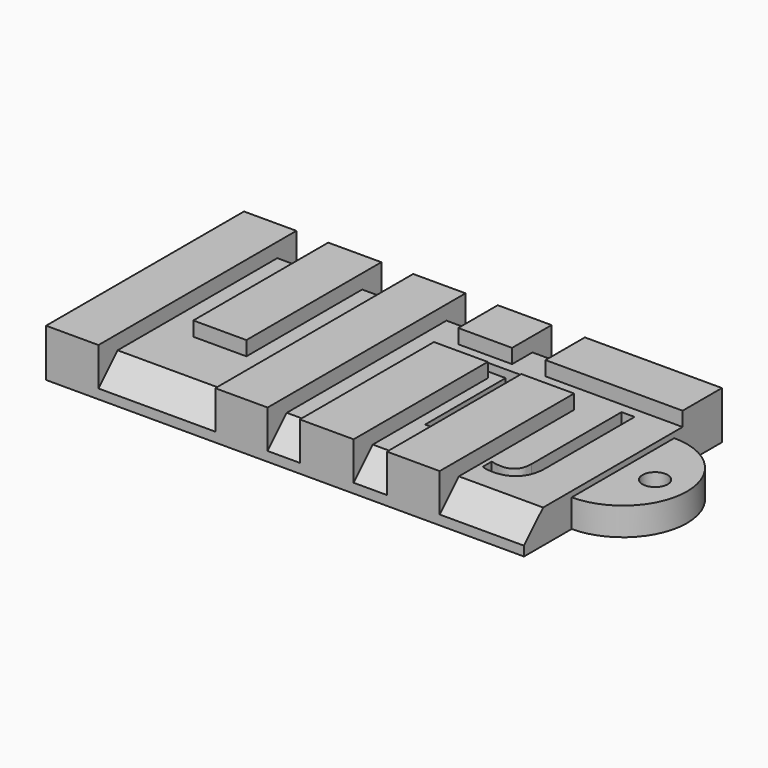
from build123d import *

# Parameters (mm, degrees)
F1_DEPTH     = 4.2
F0_W         = 6.5777550638
F0_H         = 31.0568130806
F0_W_2       = 6.6643171012
F0_H_2       = 21.1724707555
F0_W_3       = 6.5723955631
F0_W_4       = 6.7562386394
F0_H_3       = 6.1960610162
F0_H_4       = 21.0460054386
F0_W_5       = 6.6203959286
F0_H_5       = 21.0919662077
F0_W_6       = 17.2071668506
F0_H_6       = 6.1697455656
F2_DEPTH     = 6
F0_R         = 1.5875
F3_DEPTH     = 3.5
F4_TEXT_SIZE = 19.7454847188
F5_DEPTH     = 25
F6_SIZE      = 3


# Not quite as in the source:
# - Text() gives the source's letters only with a copy of the font that has no kerning and outlines rounded to 1/6400 em; it was checked with that copy


with BuildPart() as f1:
    # F0 (on Top) → F1 (new body)
    with BuildSketch(Plane.XY):
        Polygon((-63.7559369206, -7.0417550277), (-67.7545294166, -7.0417550277), (-67.7545294166, -38.0985681083), (-53.0930310488, -38.0985681083), (-53.0930310488, -7.0417550277), (-57.0916198194, -7.0417550277), (-57.0916198194, -28.2142257832), (-63.7559369206, -28.2142257832), align=None)
    extrude(amount=F1_DEPTH)



with BuildPart() as f1b:
    # F0 (on Top) → F1, piece 2 (new body)
    with BuildSketch(Plane.XY):
        Polygon((-46.5206354856, -7.0417550277), (-46.5206354856, -38.0985681083), (-42.4760840833, -38.0985681083), (-42.4760840833, -17.0525626697), (-35.719845444, -17.0525626697), (-35.719845444, -38.0985681083), (-31.5394513309, -38.0985681083), (-31.5394513309, -17.0066019006), (-24.9190554023, -17.0066019006), (-24.9190554023, -38.0985681083), (-14.3322844803, -38.0985681083), (-14.3322844803, -30.6171796859), (-14.3322844803, -14.5231434501), (-14.3322844803, -13.2115005933), (-31.5394513309, -13.2115005933), (-31.5394513309, -7.0417550277), (-35.719845444, -7.0417550277), (-35.719845444, -13.2378160439), (-42.4760840833, -13.2378160439), (-42.4760840833, -7.0417550277), align=None)
    extrude(amount=F1_DEPTH)


with BuildPart() as f1_1:
    add(f1.part)

    add(f1b.part)  # F2 merges F1b
    # F0 (on Top) → F2 (join)
    with BuildSketch(Plane.XY):
        with Locations((-71.0434069484, -22.570161568)):
            Rectangle(F0_W, F0_H)
        with Locations((-60.42377837, -17.6279904054)):
            Rectangle(F0_W_2, F0_H_2)
        with Locations((-49.8068332672, -22.570161568)):
            Rectangle(F0_W_3, F0_H)
        with Locations((-39.0979647636, -10.1397855358)):
            Rectangle(F0_W_4, F0_H_3)
        with Locations((-39.0979647636, -27.575565389)):
            Rectangle(F0_W_4, F0_H_4)
        with Locations((-28.2292533666, -27.5525850045)):
            Rectangle(F0_W_5, F0_H_5)
        with Locations((-22.9358679056, -10.1266278105)):
            Rectangle(F0_W_6, F0_H_6)
    extrude(amount=F2_DEPTH)

    # F0 (on Top) → F3 (join)
    with BuildSketch(Plane.XY):
        with BuildLine():
            Line((-14.3322844803, -14.5231434501), (-14.3322844803, -30.6171796859))
            ThreePointArc((-14.3322844803, -30.6171796859), (-6.2852663624, -22.570161568), (-14.3322844803, -14.5231434501))
        make_face()
        with Locations((-10.300190188, -22.570161568)):
            Circle(F0_R, mode=Mode.SUBTRACT)
    extrude(amount=F3_DEPTH)

    # F4 (on face) → F5 (cut)
    with BuildSketch(Plane.XY.offset(4.2)):
        with Locations((-39.0060693026, -28.5764010325)):
            Text('T', F4_TEXT_SIZE, font='Open Sans', text_align=(TextAlign.LEFT, TextAlign.BOTTOM))
        with Locations((-22.8147171438, -28.5764010325)):
            Text('J', F4_TEXT_SIZE, font='Open Sans', text_align=(TextAlign.LEFT, TextAlign.BOTTOM))
    extrude(amount=-F5_DEPTH, mode=Mode.SUBTRACT)

    # F6
    f6_edges = [f1_1.edges().sort_by_distance(p)[0] for p in [
        (-65.755233, -7.041755, 4.2),
        (-55.092325, -7.041755, 4.2),
        (-44.49836, -7.041755, 4.2),
        (-33.629648, -7.041755, 4.2),
        (-60.42378, -38.098568, 4.2),
        (-44.49836, -38.098568, 4.2),
        (-33.629648, -38.098568, 4.2),
        (-19.62567, -38.098568, 4.2),
    ]]
    chamfer(f6_edges, length=F6_SIZE)


with BuildPart() as f1_2:
    # F8: moved
    add(f1_1.part.moved(Location((44.3322844803, 22.9586008936, 0))))


solid = f1_2.part
